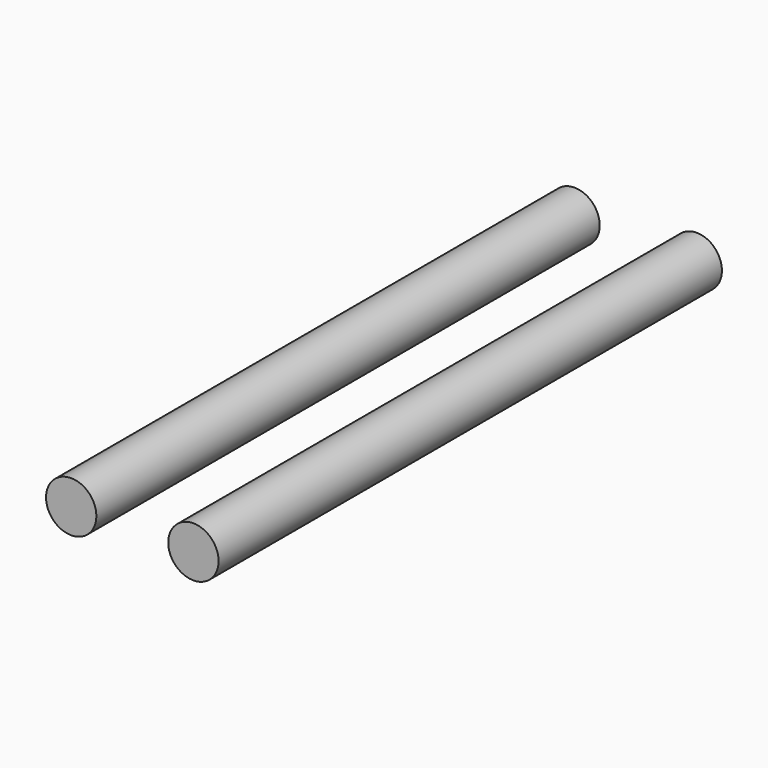
from build123d import *

# Parameters (mm, degrees)
F3_R     = 2.54
F4_DEPTH = 31.75


# Not quite as in the source:
# - the program builds the solid bodies; features that only make, move or delete a surface that nothing else refers to are left out


with BuildPart() as f4:
    # F3 (on Front) → F4 (new body, symmetric)
    with BuildSketch(Plane.XZ):
        with Locations((6.1665093526, 32.4129015207)):
            Circle(F3_R)
    extrude(amount=F4_DEPTH, both=True)


with BuildPart() as f4b:
    # F3 (on Front) → F4, piece 2 (new body, symmetric)
    with BuildSketch(Plane.XZ):
        with Locations((-6.1665093526, 32.4129015207)):
            Circle(F3_R)
    extrude(amount=F4_DEPTH, both=True)


solid = Compound([f4.part, f4b.part])
